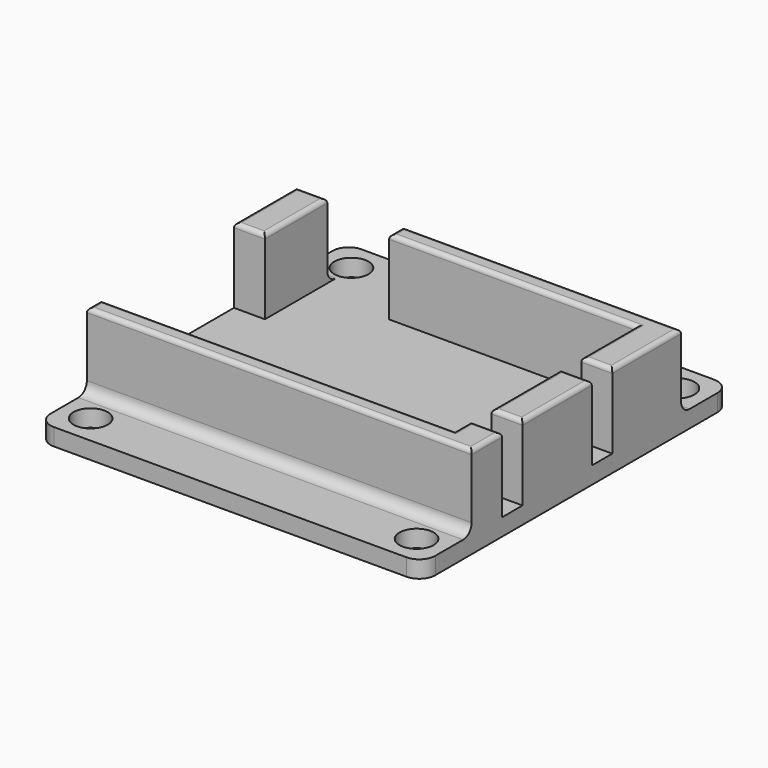
from build123d import *

# Parameters (mm, degrees)
F0_R     = 1.6
F1_DEPTH = 1.6
F2_W     = 2.9
F2_H     = 8.1
F2_H_2   = 1.65
F3_DEPTH = 7
F4_R     = 1
F5_R     = 0.4


with BuildPart() as f1:
    # F0 (on Top) → F1 (new body)
    with BuildSketch(Plane.XY):
        with BuildLine():
            ThreePointArc((-18, -16.5), (-17.5606601718, -17.5606601718), (-16.5, -18))
            Line((-16.5, -18), (16.5, -18))
            ThreePointArc((16.5, -18), (17.5606601718, -17.5606601718), (18, -16.5))
            Line((18, -16.5), (18, 16.5))
            ThreePointArc((18, 16.5), (17.5606601718, 17.5606601718), (16.5, 18))
            Line((16.5, 18), (-16.5, 18))
            ThreePointArc((-16.5, 18), (-17.5606601718, 17.5606601718), (-18, 16.5))
            Line((-18, 16.5), (-18, -16.5))
        make_face()
        with Locations((-15.25, -15.25)):
            Circle(F0_R, mode=Mode.SUBTRACT)
        with Locations((15.25, -15.25)):
            Circle(F0_R, mode=Mode.SUBTRACT)
        with Locations((-15.25, 15.25)):
            Circle(F0_R, mode=Mode.SUBTRACT)
        with Locations((15.25, 15.25)):
            Circle(F0_R, mode=Mode.SUBTRACT)
    extrude(amount=F1_DEPTH)

    # F2 (on face) → F3 (join)
    with BuildSketch(Plane.XY.offset(1.6)):
        Polygon((15.1, -10.6), (-15.1, -10.6), (-15.1, -12.25), (18, -12.25), (18, -8.7), (15.1, -8.7), align=None)
        with Locations((16.55, -2.25)):
            Rectangle(F2_W, F2_H)
        Polygon((-8, 12.25), (-8, 10.6), (15.1, 10.6), (15.1, 4.2), (18, 4.2), (18, 12.25), align=None)
        Polygon((-18, 4.95), (-15.1, 4.95), (-15.1, 10.6), (-15.1, 12.25), (-18, 12.25), align=None)
        with Locations((-16.55, -11.425)):
            Rectangle(F2_W, F2_H_2)
    extrude(amount=F3_DEPTH)

    # F4
    f4_edges = [f1.edges().sort_by_distance(p)[0] for p in [
        (0, -12.25, 1.6),
        (5, 12.25, 1.6),
        (-16.55, 12.25, 1.6),
    ]]
    fillet(f4_edges, radius=F4_R)

    # F5
    f5_edges = [f1.edges().sort_by_distance(p)[0] for p in [
        (5, 12.25, 8.6),
        (3.55, 10.6, 8.6),
        (-15.1, 8.6, 8.6),
        (-18, 8.6, 8.6),
        (-16.55, 12.25, 8.6),
        (-8, 11.425, 8.6),
        (-16.55, 4.95, 8.6),
        (-1.45, -10.6, 8.6),
        (0, -12.25, 8.6),
        (16.55, -8.7, 8.6),
        (18, -10.475, 8.6),
        (15.1, -9.65, 8.6),
        (16.55, -6.3, 8.6),
        (15.1, -2.25, 8.6),
        (18, -2.25, 8.6),
        (16.55, 1.8, 8.6),
        (16.55, 4.2, 8.6),
        (15.1, 7.4, 8.6),
        (18, 8.225, 8.6),
        (-18, -11.425, 8.6),
    ]]
    fillet(f5_edges, radius=F5_R)


solid = f1.part
